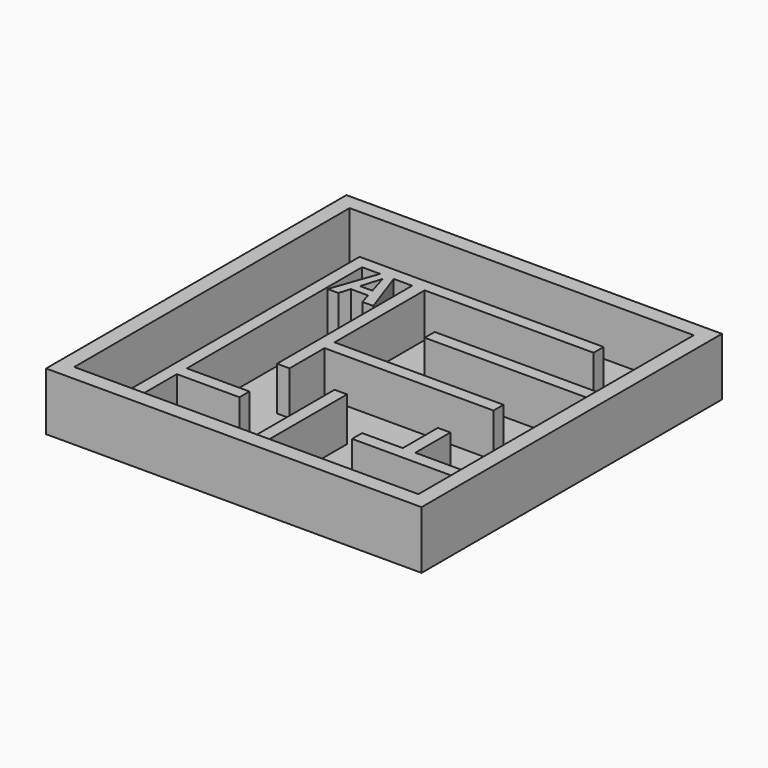
from build123d import *

# Parameters (mm, degrees)
F0_W         = 38.1
F0_H         = 38.1
F1_DEPTH     = 0.79375
F2_W         = 38.1
F2_H         = 38.1
F2_W_2       = 34.925
F2_H_2       = 34.925
F3_DEPTH     = 5.08
F4_R         = 1.27
F5_DEPTH     = 0.396875
F4_W         = 1.27
F4_H         = 10.795
F4_W_2       = 17.145
F4_H_2       = 1.27
F6_DEPTH     = 4.445
F7_TEXT_SIZE = 6.7298695922
F8_DEPTH     = 4.445


# Not quite as in the source:
# - Text() gives the source's letters only with a copy of the font that has no kerning and outlines rounded to 1/6400 em; it was checked with that copy


with BuildPart() as f1:
    # F0 (on Top) → F1 (new body)
    with BuildSketch(Plane.XY):
        with Locations((1.0833106935, 13.4667169576)):
            Rectangle(F0_W, F0_H)
    extrude(amount=F1_DEPTH)

    # F2 (on face) → F3 (join)
    with BuildSketch(Plane.XY.offset(0.79375)):
        with Locations((1.0833106935, 13.4667169576)):
            Rectangle(F2_W, F2_H)
        with Locations((1.0833106935, 13.4667169576)):
            Rectangle(F2_W_2, F2_H_2, mode=Mode.SUBTRACT)
    extrude(amount=F3_DEPTH)

    # F4 (on face) → F5 (cut)
    with BuildSketch(Plane.XY.offset(0.79375)):
        with Locations((-13.8391893065, -1.1494703705)):
            Circle(F4_R)
        with Locations((-6.709282324, -1.4557830424)):
            Circle(F4_R)
    extrude(amount=-F5_DEPTH, mode=Mode.SUBTRACT)

    # F4 (on face) → F6 (join)
    with BuildSketch(Plane.XY.offset(0.79375)):
        Polygon((-11.2991893065, 25.8492169576), (-11.2991893065, -3.9957830424), (-10.0291893065, -3.9957830424), (-10.0291893065, 1.0842169576), (-3.6791893065, 1.0842169576), (-3.6791893065, 2.3542169576), (-10.0291893065, 2.3542169576), (-10.0291893065, 24.5792169576), (-6.2191893065, 24.5792169576), (-4.9491893065, 24.5792169576), (-4.9491893065, 13.2655224284), (-4.9491893065, 7.4342169576), (-3.6791893065, 7.4342169576), (-3.6791893065, 11.8792169576), (13.4658106935, 11.8792169576), (13.4658106935, 13.1492169576), (-3.6791893065, 13.1492169576), (-3.6791893065, 13.2655224284), (-3.6791893065, 24.5792169576), (13.4658106935, 24.5792169576), (13.4658106935, 25.8492169576), (-10.0291893065, 25.8492169576), align=None)
        with Locations((2.0358106935, 1.4017169576)):
            Rectangle(F4_W, F4_H)
        Polygon((7.7508106935, 1.0842169576), (18.5458106935, 1.0842169576), (18.5458106935, 2.3542169576), (13.1483106935, 2.3542169576), (13.1483106935, 6.7992169576), (11.8783106935, 6.7992169576), (11.8783106935, 2.3542169576), (7.7508106935, 2.3542169576), align=None)
        with Locations((9.9733106935, 18.8642169576)):
            Rectangle(F4_W_2, F4_H_2)
    extrude(amount=F6_DEPTH)

    # F7 (on face) → F8 (join)
    with BuildSketch(Plane.XY.offset(0.79375)):
        with Locations((-9.8309154668, 19.9475640355)):
            Text('A', F7_TEXT_SIZE, font='Open Sans', font_style=FontStyle.BOLD, text_align=(TextAlign.LEFT, TextAlign.BOTTOM))
    extrude(amount=F8_DEPTH)


solid = f1.part
